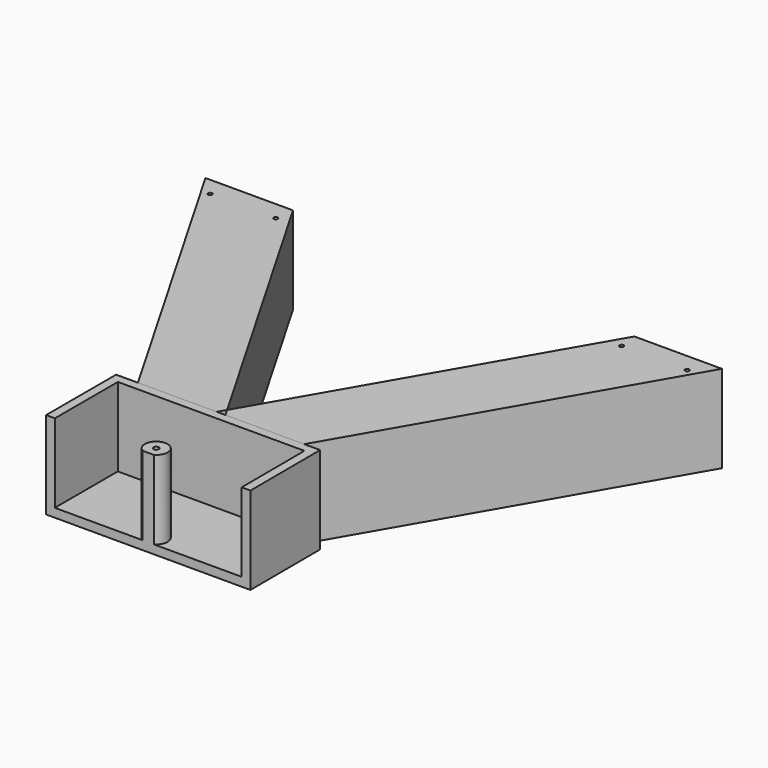
from build123d import *

# Parameters (mm, degrees)
F0_R     = 0.60325
F1_DEPTH = 25.4
F0_R_2   = 0.6096
F2_DEPTH = 25.4
F0_W     = 58.928
F0_H     = 25.1030587018
F0_R_3   = 0.762
F3_DEPTH = 25.4
F4_T     = 2.54


# Not quite as in the source:
# - a shell that OpenCascade refuses in one call is made with other operations: the cavity is built on its own and cut out


with BuildPart() as f1:
    # F0 (on Top) → F1 (new body)
    with BuildSketch(Plane.XY):
        Polygon((-74.1166336828, 65.3244355693), (-23.3166336828, -22.6637454552), (-0.4566336828, -22.6637454552), (0.8133663172, -20.4640409296), (-48.7166336828, 65.3244355693), align=None)
        with Locations((-68.3971781588, 59.8737336695)):
            Circle(F0_R, mode=Mode.SUBTRACT)
        with Locations((-49.3471781588, 59.8737336695)):
            Circle(F0_R, mode=Mode.SUBTRACT)
    extrude(amount=F1_DEPTH)


with BuildPart() as f1b:
    # F0 (on Top) → F1, piece 2 (new body)
    with BuildSketch(Plane.XY):
        Polygon((0.8133663172, -20.4640409296), (2.0833663172, -22.6637454552), (24.9433663172, -22.6637454552), (75.7433663172, 65.3244355693), (50.3433663172, 65.3244355693), align=None)
        with Locations((50.9828218412, 59.8737336695)):
            Circle(F0_R_2, mode=Mode.SUBTRACT)
        with Locations((70.0328218412, 59.8737336695)):
            Circle(F0_R_2, mode=Mode.SUBTRACT)
    extrude(amount=F1_DEPTH)


with BuildPart() as f2:
    # F0 (on Top) → F2 (new body)
    with BuildSketch(Plane.XY):
        Polygon((-23.3166336828, -22.6637454552), (-29.6483605915, -22.6637454552), (-29.6483605915, -48.0635650456), (-29.464, -48.0635650456), (-29.464, -22.9605063438), (29.464, -22.9605063438), (29.464, -48.0635650456), (29.6472443531, -48.0635650456), (29.5515115134, -22.6637454552), (24.9433663172, -22.6637454552), (2.0833663172, -22.6637454552), (-0.4566336828, -22.6637454552), align=None)
    extrude(amount=F2_DEPTH)

    # F0 (on Top) → F3 (join)
    with BuildSketch(Plane.XY):
        with Locations((0, -35.5120356947)):
            Rectangle(F0_W, F0_H)
        with Locations((0, -45.1855063438)):
            Circle(F0_R_3, mode=Mode.SUBTRACT)
    extrude(amount=F3_DEPTH)

    # F4: shell of thickness 2.54, made by hand


with BuildPart() as f4_core1:
    # F4_t2: copy of F2
    add(f2.part)

    # the walls: a layer under each face that stays
    f4_faces = [f4_core1.faces().sort_by_distance(p)[0] for p in [
        (-0.048424539, -22.6637454552, 12.7),
        (-0.0005581192, -35.3636552504, 0),
        (-0.762, -45.1855063438, 12.7),
        (-29.6483605915, -35.3636552504, 12.7),
        (29.5993779332, -35.3636552504, 12.7),
    ]]
    thicken(f4_faces, amount=-F4_T, mode=Mode.SUBTRACT)


with BuildPart() as f2_1:
    add(f2.part)

    # what is left inside the walls is the cavity
    f4_cavity = [f4_core1.part.solids().sort_by_distance(p)[0] for p in [
        (-0.043647, -25.229145, 17.78),
    ]]
    add(f4_cavity, mode=Mode.SUBTRACT)


solid = Compound([f1.part, f1b.part, f2_1.part])
